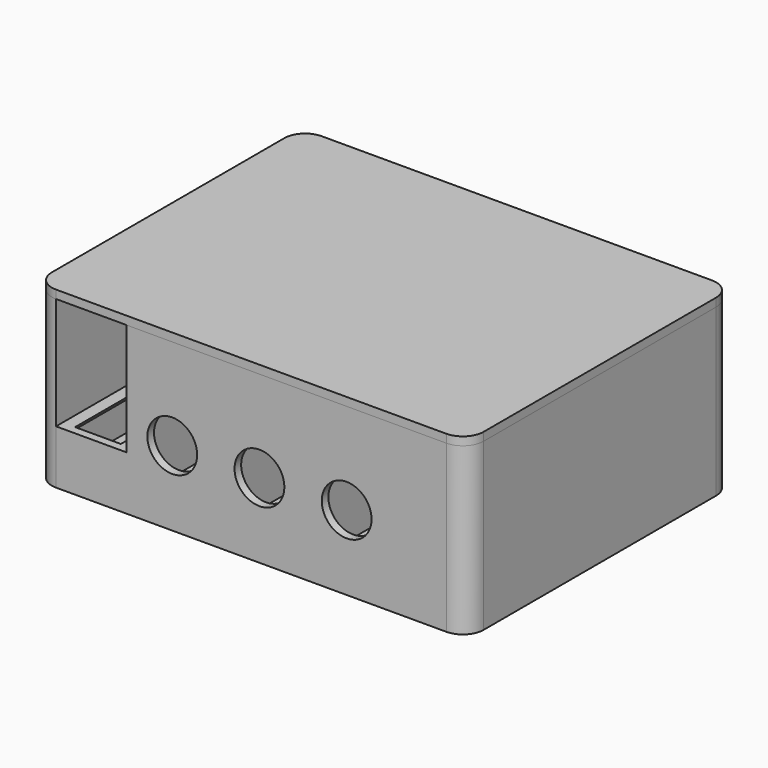
from build123d import *

# Parameters (mm, degrees)
F0_W          = 100
F0_H          = 76
F1_DEPTH      = 3
F3_W          = 104
F3_H          = 80
F3_W_2        = 100
F3_H_2        = 76
F4_DEPTH      = 40
F5_R          = 5
F6_R          = 5
F7_DEPTH      = 40
F8_R          = 6
F9_DEPTH      = 14.9
F10_W         = 12
F10_H         = 30
F11_DEPTH     = 7.1
F12_R         = 5
F13_DEPTH     = 5
F14_R         = 5.5
F14_R_2       = 3
F15_DEPTH     = 25
F16_TEXT_SIZE = 27.7777777778
F17_DEPTH     = 1
F19_DEPTH     = 32
F20_R         = 3
F21_DEPTH     = 1
F20_R_2       = 4.2
F22_DEPTH     = 8
F24_DEPTH     = 2
F25_W         = 2.17454772
F25_H         = 28.5653593019
F26_DEPTH     = 15


# Not quite as in the source:
# - Text() gives the source's letters only with a copy of the font that has no kerning and outlines rounded to 1/6400 em; it was checked with that copy


with BuildPart() as f1:
    # F0 (on Top) → F1 (new body)
    with BuildSketch(Plane.XY):
        Rectangle(F0_W, F0_H)
    extrude(amount=F1_DEPTH)

    # F3 (on face) → F4 (join)
    with BuildSketch(Plane(origin=(0, 0, 0), x_dir=(1, 0, 0), z_dir=(0, 0, -1))):
        Rectangle(F3_W, F3_H)
        Rectangle(F3_W_2, F3_H_2, mode=Mode.SUBTRACT)
    extrude(amount=-F4_DEPTH)

    # F5
    f5_edges = [f1.edges().sort_by_distance(p)[0] for p in [
        (52, -40, 20),
        (52, 40, 20),
        (-52, -40, 20),
        (-52, 40, 20),
    ]]
    fillet(f5_edges, radius=F5_R)

    # F6
    f6_edges = [f1.edges().sort_by_distance(p)[0] for p in [
        (50, 38, 21.5),
        (-50, 38, 21.5),
        (-50, -38, 21.5),
        (50, -38, 21.5),
    ]]
    fillet(f6_edges, radius=F6_R)

    # F2 (on Top) → F7 (join, through all)
    with BuildSketch(Plane.XY):
        Polygon((-48, -6), (-48, -38), (-47, -38), (-47, -8), (-30, -8), (-30, -38), (-29, -38), (-29, -12), (-9, -12), (-9, -38), (-8, -38), (-8, -12), (12, -12), (12, -38), (13, -38), (13, -12), (33, -12), (33, -38), (34, -38), (34, -10), (-29, -10), (-29, -8), (-29, -6), align=None)
    extrude(amount=F7_DEPTH)

    # F8 (on face) → F9 (cut)
    with BuildSketch(Plane.XZ.offset(40)):
        with Locations((-19, 18)):
            Circle(F8_R)
        with Locations((2, 18)):
            Circle(F8_R)
        with Locations((23, 18)):
            Circle(F8_R)
        Polygon((-47, 40.0000000001), (-47, 30), (-47, 13.0000000001), (-30, 13.0000000001), (-30, 30), (-30, 40.0000000001), align=None)
    extrude(amount=-F9_DEPTH, mode=Mode.SUBTRACT)

    # F10 (on face) → F11 (cut)
    with BuildSketch(Plane(origin=(0, -10, 0), x_dir=(-1, 0, 0), z_dir=(0, 1, 0))):
        with Locations((-23, 25)):
            Rectangle(F10_W, F10_H)
        with Locations((-2, 25)):
            Rectangle(F10_W, F10_H)
        with Locations((19, 25)):
            Rectangle(F10_W, F10_H)
    extrude(amount=-F11_DEPTH, mode=Mode.SUBTRACT)

    # F12 (on face) → F13 (cut)
    with BuildSketch(Plane(origin=(0, -6, 0), x_dir=(-1, 0, 0), z_dir=(0, 1, 0))):
        with Locations((38.5, 33.0000000001)):
            Circle(F12_R)
        with Locations((38.5, 20.0000000001)):
            Circle(F12_R)
    extrude(amount=-F13_DEPTH, mode=Mode.SUBTRACT)

    # F14 (on face) → F15 (cut)
    with BuildSketch(Plane(origin=(0, 0, 0), x_dir=(1, 0, 0), z_dir=(0, 0, -1))):
        with Locations((-27, -15)):
            Circle(F14_R)
        with Locations((27, -15)):
            Circle(F14_R)
        with Locations((44, 32)):
            Circle(F14_R_2)
    extrude(amount=-F15_DEPTH, mode=Mode.SUBTRACT)

    # F16 (on face) → F17 (cut)
    with BuildSketch(Plane(origin=(0, 0, 0), x_dir=(1, 0, 0), z_dir=(0, 0, -1))):
        with Locations((-45.6987847222, 1.4819141148)):
            Text('Brutto', F16_TEXT_SIZE, font='Open Sans', font_style=FontStyle.BOLD, text_align=(TextAlign.LEFT, TextAlign.BOTTOM))
    extrude(amount=-F17_DEPTH, mode=Mode.SUBTRACT)

    # F18 (on face) → F19 (join, through all)
    with BuildSketch(Plane.XZ.offset(40)):
        Polygon((-44, 13.0000000001), (-47, 13.0000000001), (-47, 10.0000000001), align=None)
        Polygon((-30, 10.0000000001), (-30, 13.0000000001), (-33, 13.0000000001), align=None)
    extrude(amount=-F19_DEPTH)

    # F20 (on face) → F21 (cut)
    with BuildSketch(Plane.XY.offset(3)):
        with Locations((44, -20.344336973)):
            Circle(F20_R)
    extrude(amount=-F21_DEPTH, mode=Mode.SUBTRACT)

    # F20 (on face) → F22 (join)
    with BuildSketch(Plane.XY.offset(3)):
        with Locations((44, -20.344336973)):
            Circle(F20_R_2)
        with Locations((44, -20.344336973)):
            Circle(F20_R, mode=Mode.SUBTRACT)
    extrude(amount=F22_DEPTH)


with BuildPart() as f24:
    # F23 (on face) → F24 (new body)
    with BuildSketch(Plane.XY.offset(40)):
        with BuildLine():
            ThreePointArc((-47, 40), (-50.5355339059, 38.5355339059), (-52, 35))
            Line((-52, 35), (-52, -35))
            ThreePointArc((-52, -35), (-50.5355339059, -38.5355339059), (-47, -40))
            Line((-47, -40), (-30, -40))
            Line((-30, -40), (47, -40))
            ThreePointArc((47, -40), (50.5355339059, -38.5355339059), (52, -35))
            Line((52, -35), (52, 35))
            ThreePointArc((52, 35), (50.5355339059, 38.5355339059), (47, 40))
            Line((47, 40), (-47, 40))
        make_face()
    extrude(amount=F24_DEPTH)

    # F25 (on face) → F26 (join)
    with BuildSketch(Plane.XY.offset(40)):
        with BuildLine():
            Line((34.2, -36.1237376928), (34.2, -37.8))
            Line((34.2, -37.8), (45, -37.8))
            ThreePointArc((45, -37.8), (48.3941125497, -36.3941125497), (49.8, -33))
            Line((49.8, -33), (49.8, 33))
            ThreePointArc((49.8, 33), (48.3941125497, 36.3941125497), (45, 37.8))
            Line((45, 37.8), (-30.2332527936, 37.8))
            Line((-30.2332527936, 37.8), (-30.2332527936, 35.2625176311))
            Line((-30.2332527936, 35.2625176311), (45, 35.2625176311))
            Line((45, 35.2625176311), (47.66504094, 33.0185480416))
            Line((47.66504094, 33.0185480416), (47.66504094, -33))
            Line((47.66504094, -33), (45, -36.1237376928))
            Line((45, -36.1237376928), (34.2, -36.1237376928))
        make_face()
        with Locations((-48.71272614, 16.4856924675)):
            Rectangle(F25_W, F25_H)
    extrude(amount=-F26_DEPTH)


solid = Compound([f1.part, f24.part])
